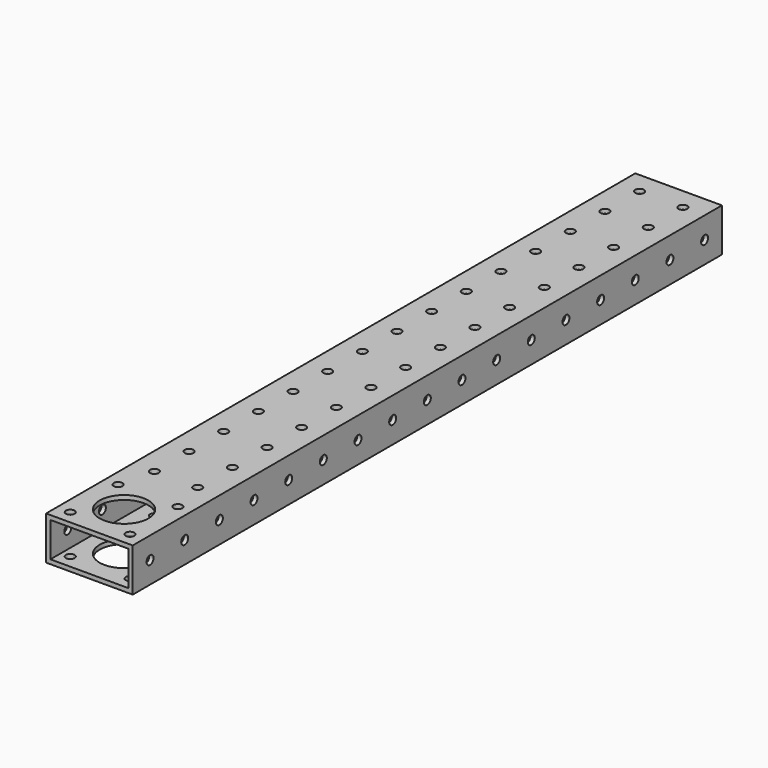
from build123d import *

# Parameters (mm, degrees)
F0_W     = 50.8
F0_H     = 431.8
F1_DEPTH = 25.4
F4_D     = 5.1054
F6_D     = 5.1054
F8_D     = 5.1054
F2_W     = 45.72
F2_H     = 20.32
F9_DEPTH = 431.8
F10_D    = 28.575


# Not quite as in the source:
# - a feature names something its author has since deleted; it is built from what else it names


with BuildPart() as f1:
    # F0 (on Top) → F1 (new body)
    with BuildSketch(Plane.XY):
        with Locations((-28.1036759261, 229.4025395081)):
            Rectangle(F0_W, F0_H)
    extrude(amount=F1_DEPTH)

    # F4 (through all)
    with Locations(Plane(origin=(-53.5036759261, 0, 0), x_dir=(0, -1, 0), z_dir=(-1, 0, 0))):
        with Locations((-26.2025395081, 12.7), (-331.0025395081, 12.7), (-381.8025395081, 12.7), (-356.4025395081, 12.7), (-407.2025395081, 12.7), (-178.6025395081, 12.7), (-229.4025395081, 12.7), (-204.0025395081, 12.7), (-280.2025395081, 12.7), (-254.8025395081, 12.7), (-305.6025395081, 12.7), (-102.4025395081, 12.7), (-153.2025395081, 12.7), (-51.6025395081, 12.7), (-127.8025395081, 12.7), (-77.0025395081, 12.7), (-432.6025395081, 12.7)):
            Hole(F4_D / 2)

    # F6 (through all)
    with Locations(Plane.XY.offset(25.4)):
        with Locations((-40.8036759261, 432.6025395081), (-15.4036759261, 432.6025395081), (-40.8036759261, 356.4025395081), (-40.8036759261, 381.8025395081), (-40.8036759261, 407.2025395081), (-40.8036759261, 254.8025395081), (-15.4036759261, 356.4025395081), (-15.4036759261, 254.8025395081), (-15.4036759261, 127.8025395081), (-40.8036759261, 102.4025395081), (-15.4036759261, 407.2025395081), (-15.4036759261, 331.0025395081), (-15.4036759261, 305.6025395081), (-40.8036759261, 204.0025395081), (-40.8036759261, 305.6025395081), (-15.4036759261, 280.2025395081), (-40.8036759261, 127.8025395081), (-15.4036759261, 381.8025395081), (-40.8036759261, 77.0025395081), (-40.8036759261, 178.6025395081), (-40.8036759261, 280.2025395081), (-15.4036759261, 77.0025395081), (-15.4036759261, 204.0025395081), (-15.4036759261, 178.6025395081), (-15.4036759261, 229.4025395081), (-15.4036759261, 153.2025395081), (-40.8036759261, 331.0025395081), (-40.8036759261, 229.4025395081), (-15.4036759261, 102.4025395081), (-40.8036759261, 153.2025395081)):
            Hole(F6_D / 2)

    # F8 (through all)
    with Locations(Plane.XY.offset(25.4)):
        with Locations((-45.6296759261, 56.4285395081), (-10.5776759261, 56.4285395081), (-10.5776759261, 21.3765395081), (-45.6296759261, 21.3765395081)):
            Hole(F8_D / 2)

    # F2 (on face) → F9 (cut)
    with BuildSketch(Plane(origin=(0, 445.3025395081, 0), x_dir=(-1, 0, 0), z_dir=(0, 1, 0))):
        with Locations((28.1036759261, 12.7)):
            Rectangle(F2_W, F2_H)
    extrude(amount=-F9_DEPTH, mode=Mode.SUBTRACT)

    # F10 (through all)
    with Locations(Plane.XY.offset(25.4)):
        with Locations((-28.1036759261, 38.9025395081)):
            Hole(F10_D / 2)


solid = f1.part
